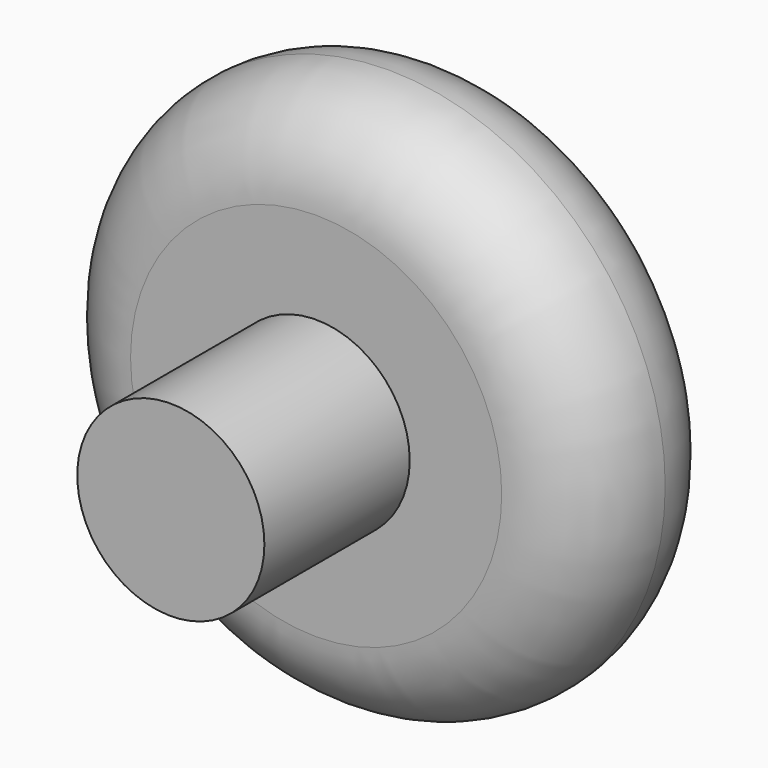
from build123d import *

# Parameters (mm, degrees)
F0_R     = 15.2162229734
F1_DEPTH = 10
F2_R     = 5.1506751803
F3_DEPTH = 10
F4_R     = 4.99999


# Not quite as in the source:
# - a fillet or chamfer is up to 0.001 mm smaller than in the source, because OpenCascade refuses the exact size


with BuildPart() as f1:
    # F0 (on Front) → F1 (new body)
    with BuildSketch(Plane.XZ):
        Circle(F0_R)
    extrude(amount=F1_DEPTH)

    # F2 (on face) → F3 (join)
    with BuildSketch(Plane.XZ.offset(10)):
        Circle(F2_R)
    extrude(amount=F3_DEPTH)

    # F4 (radius 5 in the source; OpenCascade refuses exactly that, so slightly less here)
    f4_edges = [f1.edges().sort_by_distance(p)[0] for p in [
        (15.216223, -5, 0),
        (-15.216223, 0, 0),
        (-15.216223, -10, 0),
    ]]
    fillet(f4_edges, radius=F4_R)


solid = f1.part
